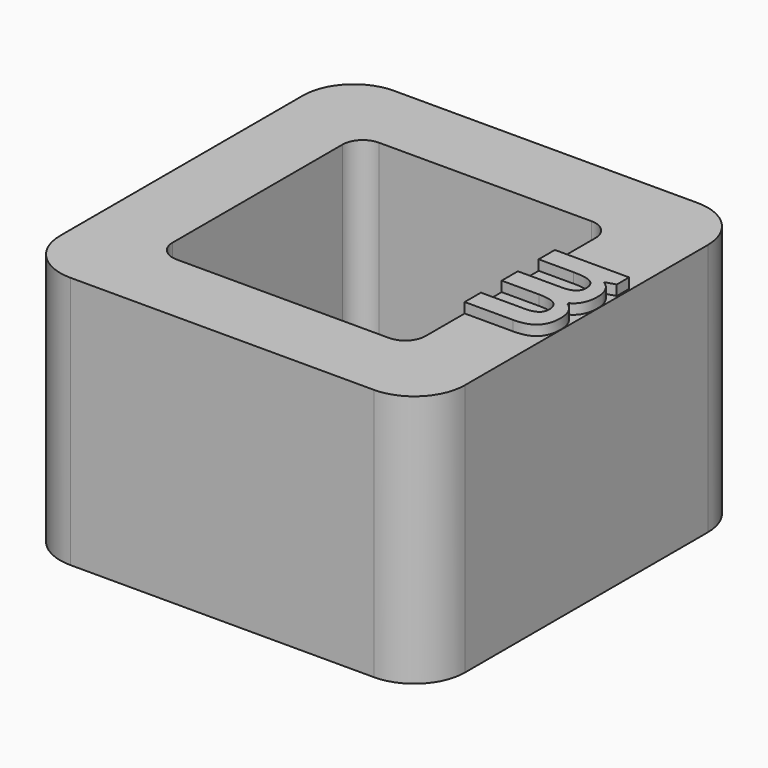
from build123d import *

# Parameters (mm, degrees)
F2_DEPTH     = 25
F1_TEXT_SIZE = 13.4389577201
F3_DEPTH     = 26


# Not quite as in the source:
# - Text() gives the source's letters only with a copy of the font that has no kerning and outlines rounded to 1/6400 em; it was checked with that copy


with BuildPart() as f2:
    # F0 (on Top) → F2 (new body)
    with BuildSketch(Plane.XY):
        with BuildLine():
            Line((15, 20), (-15, 20))
            ThreePointArc((-15, 20), (-18.5355339059, 18.5355339059), (-20, 15))
            Line((-20, 15), (-20, -15))
            ThreePointArc((-20, -15), (-18.5355339059, -18.5355339059), (-15, -20))
            Line((-15, -20), (15, -20))
            ThreePointArc((15, -20), (18.5355339059, -18.5355339059), (20, -15))
            Line((20, -15), (20, 15))
            ThreePointArc((20, 15), (18.5355339059, 18.5355339059), (15, 20))
        make_face()
        with BuildLine():
            ThreePointArc((10.5, 12.5), (11.9142135624, 11.9142135624), (12.5, 10.5))
            Line((12.5, 10.5), (12.5, -10.5))
            ThreePointArc((12.5, -10.5), (11.9142135624, -11.9142135624), (10.5, -12.5))
            Line((10.5, -12.5), (-10.5, -12.5))
            ThreePointArc((-10.5, -12.5), (-11.9142135624, -11.9142135624), (-12.5, -10.5))
            Line((-12.5, -10.5), (-12.5, 10.5))
            ThreePointArc((-12.5, 10.5), (-11.9142135624, 11.9142135624), (-10.5, 12.5))
            Line((-10.5, 12.5), (10.5, 12.5))
        make_face(mode=Mode.SUBTRACT)
    extrude(amount=F2_DEPTH)

    # F1 (on Top) → F3 (join)
    with BuildSketch(Plane.XY):
        with Locations(Location((12.5, 6.5315434357), (0, 0, -90))):
            Text('m', F1_TEXT_SIZE, font='Open Sans', font_style=FontStyle.BOLD, text_align=(TextAlign.LEFT, TextAlign.BOTTOM))
    extrude(amount=F3_DEPTH)


solid = f2.part
